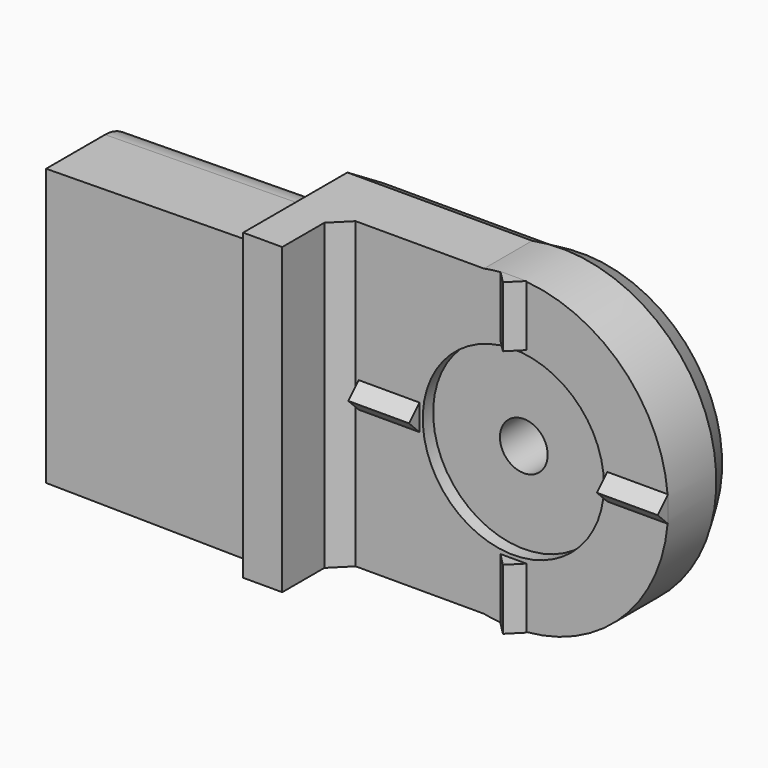
from build123d import *

# Parameters (mm, degrees)
F0_W         = 65
F0_H         = 35
F1_DEPTH     = 15
F2_R         = 17.825
F3_DEPTH     = 15
F4_W         = 39
F4_H         = 37.65
F5_DEPTH     = 8.06
F7_DEPTH     = 15.001
F8_W         = 30.8607626557
F8_H         = 37.5567990541
F9_DEPTH     = 1
F10_W        = 25.4967134297
F10_H        = 35
F11_DEPTH    = 1
F12_SIZE     = 2
F13_R        = 2.75
F14_DEPTH    = 6.941
F15_R        = 10.44
F16_DEPTH    = 1.5
F17_R        = 4.5
F19_DEPTH    = 25
F20_W        = 7
F20_H        = 3
F20_W_2      = 3
F20_H_2      = 7
F21_DEPTH    = 1.7
F22_T1_DEPTH = 15.7437221591
F22_T3_DEPTH = 15.7437221591
F22_T5_DEPTH = 11.3718610795
F22_T7_DEPTH = 15.7437221591
F3_FACE1_R   = 2.75
F23_DEPTH    = 3
F23_TAPER    = 30


# Not quite as in the source:
# - a fillet or chamfer that OpenCascade refuses, or shapes differently, is made with other operations: its cross-section is extruded or revolved along the edge and cut away or added


with BuildPart() as f1:
    # F0 (on Front) → F1 (new body)
    with BuildSketch(Plane.XZ):
        Rectangle(F0_W, F0_H)
    extrude(amount=F1_DEPTH)

    # F2 (on face) → F3 (join, through all)
    with BuildSketch(Plane.XZ.offset(15)):
        with Locations((15.675, 0)):
            Circle(F2_R)
    extrude(amount=-F3_DEPTH)

    # F4 (on face) → F5 (cut)
    with BuildSketch(Plane.XZ.offset(15)):
        with Locations((15, 0)):
            Rectangle(F4_W, F4_H)
    extrude(amount=-F5_DEPTH, mode=Mode.SUBTRACT)

    # F6 (on face) → F7 (cut, through all)
    with BuildSketch(Plane.XZ.offset(15)):
        Polygon((-9, 16.23), (-9, 17.5), (-32.5, 17.5), (-32.5, 15.93), align=None)
        Polygon((-32.5, -17.5), (-9, -17.5), (-9, -16.23), (-32.5, -15.93), align=None)
    extrude(amount=-F7_DEPTH, mode=Mode.SUBTRACT)

    # F8 (on face) → F9 (cut)
    with BuildSketch(Plane.XZ.offset(15)):
        with Locations((-24.4303813279, 1.2783995271)):
            Rectangle(F8_W, F8_H)
    extrude(amount=-F9_DEPTH, mode=Mode.SUBTRACT)

    # F10 (on face) → F11 (cut)
    with BuildSketch(Plane(origin=(0, 0, 0), x_dir=(-1, 0, 0), z_dir=(0, 1, 0))):
        with Locations((21.7483567148, 0)):
            Rectangle(F10_W, F10_H)
    extrude(amount=-F11_DEPTH, mode=Mode.SUBTRACT)

    # F12
    f12_edges = [f1.edges().sort_by_distance(p)[0] for p in [
        (-4.5, -6.94, 0),
    ]]
    chamfer(f12_edges, length=F12_SIZE)

    # F13 (on face) → F14 (cut, through all)
    with BuildSketch(Plane.XZ.offset(6.94)):
        with Locations((15.675, 0)):
            Circle(F13_R)
    extrude(amount=-F14_DEPTH, mode=Mode.SUBTRACT)

    # F15 (on face) → F16 (cut)
    with BuildSketch(Plane.XZ.offset(6.94)):
        with Locations((15.675, 0)):
            Circle(F15_R)
    extrude(amount=-F16_DEPTH, mode=Mode.SUBTRACT)

    # F17
    f17_edges = [f1.edges().sort_by_distance(p)[0] for p in [
        (-20.75, -1, 16.08),
        (-20.75, -1, -16.08),
    ]]
    fillet(f17_edges, radius=F17_R)

    # F18 (on face) → F19 (cut)
    with BuildSketch(Plane.XZ.offset(6.94)):
        with BuildLine():
            ThreePointArc((15.675, 17.825), (33.5, 0), (15.675, -17.825))
            Line((15.675, -17.825), (14.3514294177, -24.9375402927))
            Line((14.3514294177, -24.9375402927), (39.8063696921, -24.9375402927))
            Line((39.8063696921, -24.9375402927), (43.452385813, 22.5534923375))
            Line((43.452385813, 22.5534923375), (15.675, 27.0696729422))
            Line((15.675, 27.0696729422), (15.675, 17.825))
        make_face()
    extrude(amount=-F19_DEPTH, mode=Mode.SUBTRACT)

    # F20 (on face) → F21 (join)
    with BuildSketch(Plane.XZ.offset(6.94)):
        with Locations((30, 0)):
            Rectangle(F20_W, F20_H)
        with Locations((15.675, 14.325)):
            Rectangle(F20_W_2, F20_H_2)
        with Locations((1.35, 0)):
            Rectangle(F20_W, F20_H)
        with Locations((15.675, -14.325)):
            Rectangle(F20_W_2, F20_H_2)
    extrude(amount=F21_DEPTH)

    # F22: chamfer of 1.7 on 8 edges, made by hand

    # F22_s2 → F22_t1 (cut)
    with BuildSketch(Plane.YZ.offset(22.1281389205)):
        Polygon((-6.94, 1.5), (-8.64, -0.2), (-8.64, 1.5), align=None)
        Polygon((-6.94, -1.5), (-8.64, 0.2), (-8.64, -1.5), align=None)
    extrude(amount=F22_T1_DEPTH, mode=Mode.SUBTRACT)

    # F22_s4 → F22_t3 (cut)
    with BuildSketch(Plane.XY.offset(-22.1968610795)):
        Polygon((17.175, -6.94), (15.475, -8.64), (17.175, -8.64), align=None)
        Polygon((14.175, -6.94), (15.875, -8.64), (14.175, -8.64), align=None)
    extrude(amount=F22_T3_DEPTH, mode=Mode.SUBTRACT)

    # F22_s6 → F22_t5 (cut)
    with BuildSketch(Plane.YZ.offset(-2.15)):
        Polygon((-6.94, -1.5), (-8.64, 0.2), (-8.64, -1.5), align=None)
        Polygon((-6.94, 1.5), (-8.64, -0.2), (-8.64, 1.5), align=None)
    extrude(amount=F22_T5_DEPTH, mode=Mode.SUBTRACT)

    # F22_s8 → F22_t7 (cut)
    with BuildSketch(Plane.XY.offset(6.4531389205)):
        Polygon((14.175, -6.94), (15.875, -8.64), (14.175, -8.64), align=None)
        Polygon((17.175, -6.94), (15.475, -8.64), (17.175, -8.64), align=None)
    extrude(amount=F22_T7_DEPTH, mode=Mode.SUBTRACT)

    # F3_face1 (on face) → F23 (join)
    with BuildSketch(Plane(origin=(0.7743209172, 0, 0), x_dir=(-1, 0, 0), z_dir=(0, 1, 0))):
        with BuildLine():
            Line((-11.5123719834, -17.5), (9.7743209172, -17.5))
            Line((9.7743209172, -17.5), (9.7743209172, 17.5))
            Line((9.7743209172, 17.5), (-11.5123719834, 17.5))
            ThreePointArc((-11.5123719834, 17.5), (-32.7256790828, 0), (-11.5123719834, -17.5))
        make_face()
        with Locations((-14.9006790828, 0)):
            Circle(F3_FACE1_R, mode=Mode.SUBTRACT)
    extrude(amount=F23_DEPTH, taper=F23_TAPER)


solid = f1.part
